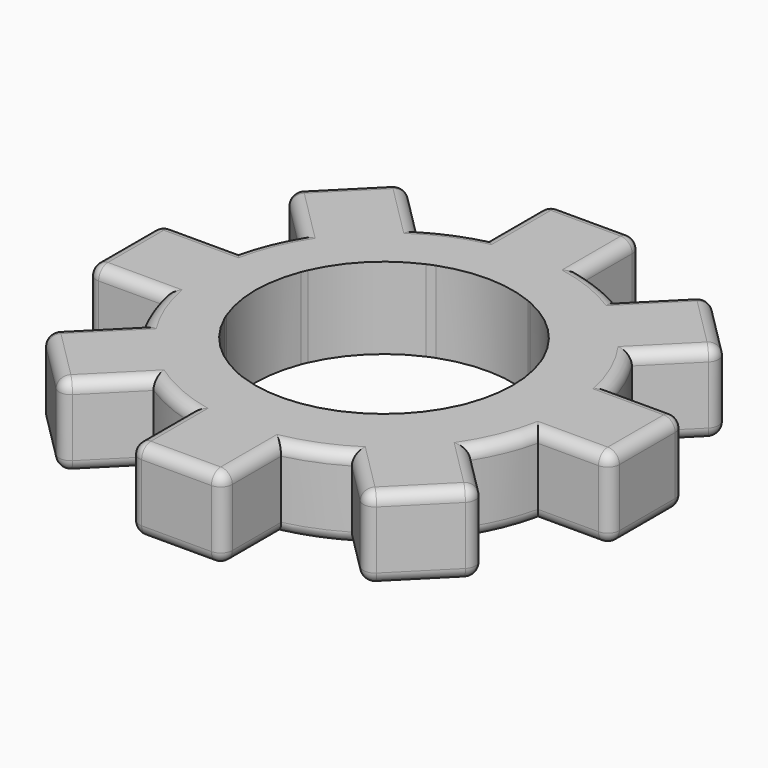
from build123d import *

# Parameters (mm, degrees)
F1_DEPTH     = 7
F2_R         = 1
F3_R         = 1
F4_T1_DEPTH  = 6
F4_T3_DEPTH  = 5
F4_T5_DEPTH  = 6
F4_T7_DEPTH  = 6
F4_T9_DEPTH  = 6
F4_T11_DEPTH = 6
F4_T13_DEPTH = 6
F4_T16_ANGLE = 90
F4_T18_ANGLE = 90
F4_T20_ANGLE = 90
F4_T22_ANGLE = 90
F4_T24_ANGLE = 90
F4_T26_ANGLE = 90
F4_T28_ANGLE = 90
F4_T30_ANGLE = 90
F4_T32_ANGLE = 90
F4_T34_ANGLE = 90
F4_T36_ANGLE = 90
F4_T38_ANGLE = 90
F4_T40_ANGLE = 90
F4_T42_ANGLE = 90
F4_T44_ANGLE = 90
F4_T46_ANGLE = 90
F4_T48_ANGLE = 90
F4_T50_ANGLE = 90
F4_T52_ANGLE = 90
F4_T54_ANGLE = 90
F4_T56_ANGLE = 90
F4_T58_ANGLE = 90
F4_T60_ANGLE = 90
F4_T62_ANGLE = 90
F4_T64_ANGLE = 90
F4_T66_ANGLE = 90
F4_T68_ANGLE = 90
F4_T70_ANGLE = 90
F4_T72_ANGLE = 90
F4_T74_ANGLE = 90
F4_T76_ANGLE = 90
F4_T78_ANGLE = 90


# Not quite as in the source:
# - a fillet or chamfer that OpenCascade refuses, or shapes differently, is made with other operations: its cross-section is extruded or revolved along the edge and cut away or added


with BuildPart() as f1:
    # F0 (on Top) → F1 (new body)
    with BuildSketch(Plane.XY):
        with BuildLine():
            Line((-18.9102605216, 13.1071560315), (-14.0960219885, 8.2929174984))
            ThreePointArc((-14.0960219885, 8.2929174984), (-11.6421815939, 11.4897849201), (-8.4893514939, 13.9999555028))
            Line((-8.4893514939, 13.9999555028), (-13.2534062721, 18.764010281))
            Line((-13.2534062721, 18.764010281), (-18.9102605216, 13.1071560315))
        make_face()
        with BuildLine():
            ThreePointArc((-8.4893514939, 13.9999555028), (-11.6421815939, 11.4897849201), (-14.0960219885, 8.2929174984))
            Line((-14.0960219885, 8.2929174984), (-10.3029473829, 4.4998428928))
            ThreePointArc((-10.3029473829, 4.4998428928), (-8.0031384218, 7.8568881812), (-4.6460931334, 10.1566971423))
            Line((-4.6460931334, 10.1566971423), (-8.4893514939, 13.9999555028))
        make_face()
        with BuildLine():
            ThreePointArc((-4, 15.9127699712), (-6.315455609, 15.1224821829), (-8.4893514939, 13.9999555028))
            Line((-8.4893514939, 13.9999555028), (-4.6460931334, 10.1566971423))
            ThreePointArc((-4.6460931334, 10.1566971423), (-4.3251030215, 10.2924612661), (-4, 10.4180581398))
            Line((-4, 10.4180581398), (-4, 15.9127699712))
        make_face()
        with BuildLine():
            ThreePointArc((4, 16.0031068635), (-0.0055323046, 16.4478649132), (-4, 15.9127699712))
            Line((-4, 15.9127699712), (-4, 10.4180581398))
            ThreePointArc((-4, 10.4180581398), (0.012449523, 11.0991456601), (4, 10.2848529747))
            Line((4, 10.2848529747), (4, 16.0031068635))
        make_face()
        with BuildLine():
            Line((-4, 22.5), (-4, 15.9127699712))
            ThreePointArc((-4, 15.9127699712), (-0.0055323046, 16.4478649132), (4, 16.0031068635))
            Line((4, 16.0031068635), (4, 22.5))
            Line((4, 22.5), (-4, 22.5))
        make_face()
        with BuildLine():
            Line((4.3022314931, 10.1566971423), (8.4085999773, 14.2630656264))
            ThreePointArc((8.4085999773, 14.2630656264), (6.2668160064, 15.2914779593), (4, 16.0031068635))
            Line((4, 16.0031068635), (4, 10.2848529747))
            ThreePointArc((4, 10.2848529747), (4.1515906147, 10.2218949458), (4.3022314931, 10.1566971423))
        make_face()
        with BuildLine():
            Line((9.9590857426, 4.4998428928), (14.1911468506, 8.7319040008))
            ThreePointArc((14.1911468506, 8.7319040008), (11.63867014, 11.8516794804), (8.4085999773, 14.2630656264))
            Line((8.4085999773, 14.2630656264), (4.3022314931, 10.1566971423))
            ThreePointArc((4.3022314931, 10.1566971423), (7.6592767815, 7.8568881812), (9.9590857426, 4.4998428928))
        make_face()
        with BuildLine():
            ThreePointArc((8.4085999773, 14.2630656264), (11.63867014, 11.8516794804), (14.1911468506, 8.7319040008))
            Line((14.1911468506, 8.7319040008), (18.5663988813, 13.1071560315))
            Line((18.5663988813, 13.1071560315), (12.9095446318, 18.764010281))
            Line((12.9095446318, 18.764010281), (8.4085999773, 14.2630656264))
        make_face()
        with BuildLine():
            Line((10.1654000803, 4), (16.2348496569, 4))
            ThreePointArc((16.2348496569, 4), (15.3980605169, 6.4458801364), (14.1911468506, 8.7319040008))
            Line((14.1911468506, 8.7319040008), (9.9590857426, 4.4998428928))
            ThreePointArc((9.9590857426, 4.4998428928), (10.0652940332, 4.2511808224), (10.1654000803, 4))
        make_face()
        with BuildLine():
            Line((10.1455068885, -4), (16.2975573812, -4))
            ThreePointArc((16.2975573812, -4), (16.6414561301, -2.0765917699), (16.7566225123, -0.126078434))
            ThreePointArc((16.7566225123, -0.126078434), (16.6256619327, 1.9533908587), (16.2348496569, 4))
            Line((16.2348496569, 4), (10.1654000803, 4))
            ThreePointArc((10.1654000803, 4), (10.7170903646, 2.0467799435), (10.9030691799, 0.0256805796))
            ThreePointArc((10.9030691799, 0.0256805796), (10.7120309499, -2.0224896254), (10.1455068885, -4))
        make_face()
        with BuildLine():
            ThreePointArc((16.7566225123, -0.126078434), (16.6414561301, -2.0765917699), (16.2975573812, -4))
            Line((16.2975573812, -4), (22.5, -4))
            Line((22.5, -4), (22.5, 4))
            Line((22.5, 4), (16.2348496569, 4))
            ThreePointArc((16.2348496569, 4), (16.6256619327, 1.9533908587), (16.7566225123, -0.126078434))
        make_face()
        with BuildLine():
            Line((9.9590857426, -4.4484817337), (14.3076564491, -8.7970524402))
            ThreePointArc((14.3076564491, -8.7970524402), (15.4916550838, -6.4769466942), (16.2975573812, -4))
            Line((16.2975573812, -4), (10.1455068885, -4))
            ThreePointArc((10.1455068885, -4), (10.0547550795, -4.2252629053), (9.9590857426, -4.4484817337))
        make_face()
        with BuildLine():
            Line((4.3022314931, -10.1053359832), (8.6006184447, -14.4037229347))
            ThreePointArc((8.6006184447, -14.4037229347), (11.7974858663, -11.9498825401), (14.3076564491, -8.7970524402))
            Line((14.3076564491, -8.7970524402), (9.9590857426, -4.4484817337))
            ThreePointArc((9.9590857426, -4.4484817337), (7.6592767815, -7.8055270221), (4.3022314931, -10.1053359832))
        make_face()
        with BuildLine():
            ThreePointArc((14.3076564491, -8.7970524402), (11.7974858663, -11.9498825401), (8.6006184447, -14.4037229347))
            Line((8.6006184447, -14.4037229347), (12.9095446318, -18.7126491219))
            Line((12.9095446318, -18.7126491219), (18.5663988813, -13.0557948724))
            Line((18.5663988813, -13.0557948724), (14.3076564491, -8.7970524402))
        make_face()
        with BuildLine():
            ThreePointArc((-4, -16.1649268392), (-0.0055323046, -16.7000217811), (4, -16.2552637315))
            Line((4, -16.2552637315), (4, -10.2334918155))
            ThreePointArc((4, -10.2334918155), (0.012449523, -11.0477845009), (-4, -10.3666969806))
            Line((-4, -10.3666969806), (-4, -16.1649268392))
        make_face()
        with BuildLine():
            Line((-4, -22.5), (4, -22.5))
            Line((4, -22.5), (4, -16.2552637315))
            ThreePointArc((4, -16.2552637315), (-0.0055323046, -16.7000217811), (-4, -16.1649268392))
            Line((-4, -16.1649268392), (-4, -22.5))
        make_face()
        with BuildLine():
            Line((4, -10.2334918155), (4, -16.2552637315))
            ThreePointArc((4, -16.2552637315), (6.369948448, -15.5025294911), (8.6006184447, -14.4037229347))
            Line((8.6006184447, -14.4037229347), (4.3022314931, -10.1053359832))
            ThreePointArc((4.3022314931, -10.1053359832), (4.1515906147, -10.1705337867), (4, -10.2334918155))
        make_face()
        with BuildLine():
            ThreePointArc((-8.6763599225, -14.1356027723), (-6.4166623661, -15.3311191003), (-4, -16.1649268392))
            Line((-4, -16.1649268392), (-4, -10.3666969806))
            ThreePointArc((-4, -10.3666969806), (-4.3251030215, -10.241100107), (-4.6460931334, -10.1053359832))
            Line((-4.6460931334, -10.1053359832), (-8.6763599225, -14.1356027723))
        make_face()
        with BuildLine():
            ThreePointArc((-14.2075215481, -8.3530558989), (-11.7961354021, -11.5831260617), (-8.6763599225, -14.1356027723))
            Line((-8.6763599225, -14.1356027723), (-4.6460931334, -10.1053359832))
            ThreePointArc((-4.6460931334, -10.1053359832), (-8.0031384218, -7.8055270221), (-10.3029473829, -4.4484817337))
            Line((-10.3029473829, -4.4484817337), (-14.2075215481, -8.3530558989))
        make_face()
        with BuildLine():
            Line((-13.2534062721, -18.7126491219), (-8.6763599225, -14.1356027723))
            ThreePointArc((-8.6763599225, -14.1356027723), (-11.7961354021, -11.5831260617), (-14.2075215481, -8.3530558989))
            Line((-14.2075215481, -8.3530558989), (-18.9102605216, -13.0557948724))
            Line((-18.9102605216, -13.0557948724), (-13.2534062721, -18.7126491219))
        make_face()
        with BuildLine():
            ThreePointArc((-15.9343123567, -4), (-15.2254289265, -6.2378204904), (-14.2075215481, -8.3530558989))
            Line((-14.2075215481, -8.3530558989), (-10.3029473829, -4.4484817337))
            ThreePointArc((-10.3029473829, -4.4484817337), (-10.3986167197, -4.2252629053), (-10.4893685287, -4))
            Line((-10.4893685287, -4), (-15.9343123567, -4))
        make_face()
        with BuildLine():
            ThreePointArc((-15.8716046323, 4), (-16.3928683144, 0.0038401412), (-15.9343123567, -4))
            Line((-15.9343123567, -4), (-10.4893685287, -4))
            ThreePointArc((-10.4893685287, -4), (-11.2468965796, -0.0018589727), (-10.5092617205, 4))
            Line((-10.5092617205, 4), (-15.8716046323, 4))
        make_face()
        with BuildLine():
            Line((-22.5, -4), (-15.9343123567, -4))
            ThreePointArc((-15.9343123567, -4), (-16.3928683144, 0.0038401412), (-15.8716046323, 4))
            Line((-15.8716046323, 4), (-22.5, 4))
            Line((-22.5, 4), (-22.5, -4))
        make_face()
        with BuildLine():
            ThreePointArc((-14.0960219885, 8.2929174984), (-15.1349609466, 6.2089745371), (-15.8716046323, 4))
            Line((-15.8716046323, 4), (-10.5092617205, 4))
            ThreePointArc((-10.5092617205, 4), (-10.4091556734, 4.2511808224), (-10.3029473829, 4.4998428928))
            Line((-10.3029473829, 4.4998428928), (-14.0960219885, 8.2929174984))
        make_face()
    extrude(amount=F1_DEPTH)

    # F2
    f2_edges = [f1.edges().sort_by_distance(p)[0] for p in [
        (-10.871379, 16.381983, 7),
        (-6.315456, 15.122482, 7),
        (-4, 19.206385, 7),
        (4, 19.251553, 7),
        (6.266816, 15.291478, 7),
        (10.659072, 16.513538, 7),
        (16.378773, 10.91953, 7),
        (19.367425, 4, 7),
        (19.398779, -4, 7),
        (15.398061, 6.44588, 7),
        (15.491655, -6.476947, 7),
        (16.437028, -10.926424, 7),
        (10.755082, -16.558186, 7),
        (6.369948, -15.502529, 7),
        (4, -19.377632, 7),
        (-4, -19.332463, 7),
        (-6.416662, -15.331119, 7),
        (-10.964883, -16.424126, 7),
        (-16.558891, -10.704425, 7),
        (-15.225429, -6.23782, 7),
        (-19.217156, -4, 7),
        (-19.185802, 4, 7),
        (-15.134961, 6.208975, 7),
        (-16.503141, 10.700037, 7),
    ]]
    fillet(f2_edges, radius=F2_R)

    # F3
    f3_edges = [f1.edges().sort_by_distance(p)[0] for p in [
        (16.437028, -10.926424, 0),
        (10.755082, -16.558186, 0),
        (15.491655, -6.476947, 0),
        (6.369948, -15.502529, 0),
        (4, -19.377632, 0),
        (-4, -19.332463, 0),
        (-6.416662, -15.331119, 0),
        (-10.964883, -16.424126, 0),
        (-16.558891, -10.704425, 0),
        (-15.225429, -6.23782, 0),
        (-19.217156, -4, 0),
        (-19.185802, 4, 0),
        (-15.134961, 6.208975, 0),
        (-16.503141, 10.700037, 0),
        (-10.871379, 16.381983, 0),
        (-6.315456, 15.122482, 0),
        (-4, 19.206385, 0),
        (4, 19.251553, 0),
        (6.266816, 15.291478, 0),
        (10.659072, 16.513538, 0),
        (16.378773, 10.91953, 0),
        (15.398061, 6.44588, 0),
        (19.367425, 4, 0),
        (19.398779, -4, 0),
    ]]
    fillet(f3_edges, radius=F3_R)

    # F4: fillet of radius 1 on 64 edges, made by hand

    # F4_s2 → F4_t1 (cut)
    with BuildSketch(Plane(origin=(-2.1944454638, -2.1944454638, 0), x_dir=(0, 0, 1), z_dir=(0.7071067812, 0.7071067812, 0))):
        with BuildLine():
            ThreePointArc((7, 21.3602676392), (6.7071067812, 22.0673744204), (6, 22.3602676392))
            Line((6, 22.3602676392), (7, 22.3602676392))
            Line((7, 22.3602676392), (7, 21.3602676392))
        make_face()
        with BuildLine():
            ThreePointArc((0, 21.3602676392), (0.2928932188, 22.0673744204), (1, 22.3602676392))
            Line((1, 22.3602676392), (0, 22.3602676392))
            Line((0, 22.3602676392), (0, 21.3602676392))
        make_face()
    extrude(amount=F4_T1_DEPTH, mode=Mode.SUBTRACT)

    # F4_s4 → F4_t3 (cut)
    with BuildSketch(Plane.XY.offset(1)):
        with BuildLine():
            ThreePointArc((13.616651413, -18.0055423407), (12.9095446318, -18.2984355595), (12.2024378507, -18.0055423407))
            Line((12.2024378507, -18.0055423407), (12.9095446318, -18.7126491219))
            Line((12.9095446318, -18.7126491219), (13.616651413, -18.0055423407))
        make_face()
        with BuildLine():
            ThreePointArc((17.8592921001, -13.7629016536), (18.152185319, -13.0557948724), (17.8592921001, -12.3486880912))
            Line((17.8592921001, -12.3486880912), (18.5663988813, -13.0557948724))
            Line((18.5663988813, -13.0557948724), (17.8592921001, -13.7629016536))
        make_face()
        with BuildLine():
            ThreePointArc((-3, -22.5), (-3.7071067812, -22.2071067812), (-4, -21.5))
            Line((-4, -21.5), (-4, -22.5))
            Line((-4, -22.5), (-3, -22.5))
        make_face()
        with BuildLine():
            ThreePointArc((3, -22.5), (3.7071067812, -22.2071067812), (4, -21.5))
            Line((4, -21.5), (4, -22.5))
            Line((4, -22.5), (3, -22.5))
        make_face()
        with BuildLine():
            ThreePointArc((-13.9605130533, -18.0055423407), (-13.2534062721, -18.2984355595), (-12.5462994909, -18.0055423407))
            Line((-12.5462994909, -18.0055423407), (-13.2534062721, -18.7126491219))
            Line((-13.2534062721, -18.7126491219), (-13.9605130533, -18.0055423407))
        make_face()
        with BuildLine():
            ThreePointArc((-18.2031537404, -13.7629016536), (-18.4960469592, -13.0557948724), (-18.2031537404, -12.3486880912))
            Line((-18.2031537404, -12.3486880912), (-18.9102605216, -13.0557948724))
            Line((-18.9102605216, -13.0557948724), (-18.2031537404, -13.7629016536))
        make_face()
        with BuildLine():
            ThreePointArc((-22.5, 3), (-22.2071067812, 3.7071067812), (-21.5, 4))
            Line((-21.5, 4), (-22.5, 4))
            Line((-22.5, 4), (-22.5, 3))
        make_face()
        with BuildLine():
            ThreePointArc((-22.5, -3), (-22.2071067812, -3.7071067812), (-21.5, -4))
            Line((-21.5, -4), (-22.5, -4))
            Line((-22.5, -4), (-22.5, -3))
        make_face()
        with BuildLine():
            ThreePointArc((-18.2031537404, 13.8142628127), (-18.4960469592, 13.1071560315), (-18.2031537404, 12.4000492503))
            Line((-18.2031537404, 12.4000492503), (-18.9102605216, 13.1071560315))
            Line((-18.9102605216, 13.1071560315), (-18.2031537404, 13.8142628127))
        make_face()
        with BuildLine():
            ThreePointArc((-13.9605130532, 18.0569034998), (-13.2534062721, 18.3497967186), (-12.5462994909, 18.0569034998))
            Line((-12.5462994909, 18.0569034998), (-13.2534062721, 18.764010281))
            Line((-13.2534062721, 18.764010281), (-13.9605130532, 18.0569034998))
        make_face()
        with BuildLine():
            ThreePointArc((3, 22.5), (3.7071067812, 22.2071067812), (4, 21.5))
            Line((4, 21.5), (4, 22.5))
            Line((4, 22.5), (3, 22.5))
        make_face()
        with BuildLine():
            ThreePointArc((-3, 22.5), (-3.7071067812, 22.2071067812), (-4, 21.5))
            Line((-4, 21.5), (-4, 22.5))
            Line((-4, 22.5), (-3, 22.5))
        make_face()
        with BuildLine():
            ThreePointArc((17.8592921001, 13.8142628127), (18.152185319, 13.1071560315), (17.8592921001, 12.4000492503))
            Line((17.8592921001, 12.4000492503), (18.5663988813, 13.1071560315))
            Line((18.5663988813, 13.1071560315), (17.8592921001, 13.8142628127))
        make_face()
        with BuildLine():
            ThreePointArc((13.616651413, 18.0569034998), (12.9095446318, 18.3497967186), (12.2024378507, 18.0569034998))
            Line((12.2024378507, 18.0569034998), (12.9095446318, 18.764010281))
            Line((12.9095446318, 18.764010281), (13.616651413, 18.0569034998))
        make_face()
        with BuildLine():
            ThreePointArc((22.5, 3), (22.2071067812, 3.7071067812), (21.5, 4))
            Line((21.5, 4), (22.5, 4))
            Line((22.5, 4), (22.5, 3))
        make_face()
        with BuildLine():
            ThreePointArc((22.5, -3), (22.2071067812, -3.7071067812), (21.5, -4))
            Line((21.5, -4), (22.5, -4))
            Line((22.5, -4), (22.5, -3))
        make_face()
    extrude(amount=F4_T3_DEPTH, mode=Mode.SUBTRACT)

    # F4_s6 → F4_t5 (cut)
    with BuildSketch(Plane.YZ.offset(-3)):
        with BuildLine():
            ThreePointArc((-21.5, 7), (-22.2071067812, 6.7071067812), (-22.5, 6))
            Line((-22.5, 6), (-22.5, 7))
            Line((-22.5, 7), (-21.5, 7))
        make_face()
        with BuildLine():
            ThreePointArc((-21.5, 0), (-22.2071067812, 0.2928932188), (-22.5, 1))
            Line((-22.5, 1), (-22.5, 0))
            Line((-22.5, 0), (-21.5, 0))
        make_face()
        with BuildLine():
            ThreePointArc((21.5, 7), (22.2071067812, 6.7071067812), (22.5, 6))
            Line((22.5, 6), (22.5, 7))
            Line((22.5, 7), (21.5, 7))
        make_face()
        with BuildLine():
            ThreePointArc((21.5, 0), (22.2071067812, 0.2928932188), (22.5, 1))
            Line((22.5, 1), (22.5, 0))
            Line((22.5, 0), (21.5, 0))
        make_face()
    extrude(amount=F4_T5_DEPTH, mode=Mode.SUBTRACT)

    # F4_s8 → F4_t7 (cut)
    with BuildSketch(Plane(origin=(-2.2201260434, 2.2201260434, 0), x_dir=(0, 0, 1), z_dir=(0.7071067812, -0.7071067812, 0))):
        with BuildLine():
            ThreePointArc((7, 21.6034145368), (6.7071067812, 22.310521318), (6, 22.6034145368))
            Line((6, 22.6034145368), (7, 22.6034145368))
            Line((7, 22.6034145368), (7, 21.6034145368))
        make_face()
        with BuildLine():
            ThreePointArc((0, 21.6034145368), (0.2928932188, 22.310521318), (1, 22.6034145368))
            Line((1, 22.6034145368), (0, 22.6034145368))
            Line((0, 22.6034145368), (0, 21.6034145368))
        make_face()
    extrude(amount=F4_T7_DEPTH, mode=Mode.SUBTRACT)

    # F4_s10 → F4_t9 (cut)
    with BuildSketch(Plane.XZ.offset(-3)):
        with BuildLine():
            ThreePointArc((-21.5, 7), (-22.2071067812, 6.7071067812), (-22.5, 6))
            Line((-22.5, 6), (-22.5, 7))
            Line((-22.5, 7), (-21.5, 7))
        make_face()
        with BuildLine():
            ThreePointArc((-21.5, 0), (-22.2071067812, 0.2928932188), (-22.5, 1))
            Line((-22.5, 1), (-22.5, 0))
            Line((-22.5, 0), (-21.5, 0))
        make_face()
        with BuildLine():
            ThreePointArc((21.5, 0), (22.2071067812, 0.2928932188), (22.5, 1))
            Line((22.5, 1), (22.5, 0))
            Line((22.5, 0), (21.5, 0))
        make_face()
        with BuildLine():
            ThreePointArc((21.5, 7), (22.2071067812, 6.7071067812), (22.5, 6))
            Line((22.5, 6), (22.5, 7))
            Line((22.5, 7), (21.5, 7))
        make_face()
    extrude(amount=F4_T9_DEPTH, mode=Mode.SUBTRACT)

    # F4_s12 → F4_t11 (cut)
    with BuildSketch(Plane(origin=(2.0481952233, 2.0481952233, 0), x_dir=(0, 0, 1), z_dir=(-0.7071067812, -0.7071067812, 0))):
        with BuildLine():
            ThreePointArc((6, 22.6397323608), (6.7071067812, 22.3468391419), (7, 21.6397323608))
            Line((7, 21.6397323608), (7, 22.6397323608))
            Line((7, 22.6397323608), (6, 22.6397323608))
        make_face()
        with BuildLine():
            ThreePointArc((1, 22.6397323608), (0.2928932188, 22.3468391419), (0, 21.6397323608))
            Line((0, 21.6397323608), (0, 22.6397323608))
            Line((0, 22.6397323608), (1, 22.6397323608))
        make_face()
    extrude(amount=F4_T11_DEPTH, mode=Mode.SUBTRACT)

    # F4_s14 → F4_t13 (cut)
    with BuildSketch(Plane(origin=(2.0225146437, -2.0225146437, 0), x_dir=(0, 0, 1), z_dir=(-0.7071067812, 0.7071067812, 0))):
        with BuildLine():
            ThreePointArc((0, 21.3965854632), (0.2928932188, 22.1036922443), (1, 22.3965854632))
            Line((1, 22.3965854632), (0, 22.3965854632))
            Line((0, 22.3965854632), (0, 21.3965854632))
        make_face()
        with BuildLine():
            ThreePointArc((7, 21.3965854632), (6.7071067812, 22.1036922443), (6, 22.3965854632))
            Line((6, 22.3965854632), (7, 22.3965854632))
            Line((7, 22.3965854632), (7, 21.3965854632))
        make_face()
    extrude(amount=F4_T13_DEPTH, mode=Mode.SUBTRACT)

    # F4_s15 → F4_t16 (revolve, cut)
    with BuildSketch(Plane.XY.offset(1)):
        with BuildLine():
            ThreePointArc((-13.9605130532, 18.0569034998), (-13.2534062721, 18.3497967186), (-12.5462994909, 18.0569034998))
            Line((-12.5462994909, 18.0569034998), (-13.2534062721, 18.764010281))
            Line((-13.2534062721, 18.764010281), (-13.9605130532, 18.0569034998))
        make_face()
    revolve(axis=Axis((-13.9605130533, 18.0569034998, 1), (-0.7071067812, 0.7071067812, 0)), revolution_arc=F4_T16_ANGLE, mode=Mode.SUBTRACT)

    # F4_s17 → F4_t18 (revolve, cut)
    with BuildSketch(Plane.XY.offset(6)):
        with BuildLine():
            ThreePointArc((-13.9605130532, 18.0569034998), (-13.2534062721, 18.3497967186), (-12.5462994909, 18.0569034998))
            Line((-12.5462994909, 18.0569034998), (-13.2534062721, 18.764010281))
            Line((-13.2534062721, 18.764010281), (-13.9605130532, 18.0569034998))
        make_face()
    revolve(axis=Axis((-13.9605130533, 18.0569034998, 6), (0.7071067812, -0.7071067812, 0)), revolution_arc=F4_T18_ANGLE, mode=Mode.SUBTRACT)

    # F4_s19 → F4_t20 (revolve, cut)
    with BuildSketch(Plane(origin=(-2.1944454638, -2.1944454638, 0), x_dir=(0, 0, 1), z_dir=(0.7071067812, 0.7071067812, 0))):
        with BuildLine():
            ThreePointArc((1, -22.6397323608), (0.2928932188, -22.3468391419), (0, -21.6397323608))
            Line((0, -21.6397323608), (0, -22.6397323608))
            Line((0, -22.6397323608), (1, -22.6397323608))
        make_face()
    revolve(axis=Axis((-18.2031537404, 13.8142628127, 1), (-0.7071067812, 0.7071067812, 0)), revolution_arc=F4_T20_ANGLE, mode=Mode.SUBTRACT)

    # F4_s21 → F4_t22 (revolve, cut)
    with BuildSketch(Plane.XY.offset(6)):
        with BuildLine():
            ThreePointArc((-18.2031537404, 13.8142628127), (-18.4960469592, 13.1071560315), (-18.2031537404, 12.4000492503))
            Line((-18.2031537404, 12.4000492503), (-18.9102605216, 13.1071560315))
            Line((-18.9102605216, 13.1071560315), (-18.2031537404, 13.8142628127))
        make_face()
    revolve(axis=Axis((-18.2031537404, 13.8142628127, 6), (-0.7071067812, 0.7071067812, 0)), revolution_arc=F4_T22_ANGLE, mode=Mode.SUBTRACT)

    # F4_s23 → F4_t24 (revolve, cut)
    with BuildSketch(Plane.YZ.offset(-3)):
        with BuildLine():
            ThreePointArc((21.5, 0), (22.2071067812, 0.2928932188), (22.5, 1))
            Line((22.5, 1), (22.5, 0))
            Line((22.5, 0), (21.5, 0))
        make_face()
    revolve(axis=Axis((-3, 22.5, 1), (0, 1, 0)), revolution_arc=F4_T24_ANGLE, mode=Mode.SUBTRACT)

    # F4_s25 → F4_t26 (revolve, cut)
    with BuildSketch(Plane.XZ.offset(-3)):
        with BuildLine():
            ThreePointArc((-21.5, 0), (-22.2071067812, 0.2928932188), (-22.5, 1))
            Line((-22.5, 1), (-22.5, 0))
            Line((-22.5, 0), (-21.5, 0))
        make_face()
    revolve(axis=Axis((-22.5, 3, 1), (1, 0, 0)), revolution_arc=F4_T26_ANGLE, mode=Mode.SUBTRACT)

    # F4_s27 → F4_t28 (revolve, cut)
    with BuildSketch(Plane.YZ.offset(3)):
        with BuildLine():
            ThreePointArc((22.5, 1), (22.2071067812, 0.2928932188), (21.5, 0))
            Line((21.5, 0), (22.5, 0))
            Line((22.5, 0), (22.5, 1))
        make_face()
    revolve(axis=Axis((3, 22.5, 1), (0, -1, 0)), revolution_arc=F4_T28_ANGLE, mode=Mode.SUBTRACT)

    # F4_s29 → F4_t30 (revolve, cut)
    with BuildSketch(Plane.XY.offset(6)):
        with BuildLine():
            ThreePointArc((3, 22.5), (3.7071067812, 22.2071067812), (4, 21.5))
            Line((4, 21.5), (4, 22.5))
            Line((4, 22.5), (3, 22.5))
        make_face()
    revolve(axis=Axis((3, 22.5, 6), (0, -1, 0)), revolution_arc=F4_T30_ANGLE, mode=Mode.SUBTRACT)

    # F4_s31 → F4_t32 (revolve, cut)
    with BuildSketch(Plane.XY.offset(6)):
        with BuildLine():
            ThreePointArc((-3, 22.5), (-3.7071067812, 22.2071067812), (-4, 21.5))
            Line((-4, 21.5), (-4, 22.5))
            Line((-4, 22.5), (-3, 22.5))
        make_face()
    revolve(axis=Axis((-3, 22.5, 6), (0, 1, 0)), revolution_arc=F4_T32_ANGLE, mode=Mode.SUBTRACT)

    # F4_s33 → F4_t34 (revolve, cut)
    with BuildSketch(Plane.XY.offset(6)):
        with BuildLine():
            ThreePointArc((-22.5, 3), (-22.2071067812, 3.7071067812), (-21.5, 4))
            Line((-21.5, 4), (-22.5, 4))
            Line((-22.5, 4), (-22.5, 3))
        make_face()
    revolve(axis=Axis((-22.5, 3, 6), (1, 0, 0)), revolution_arc=F4_T34_ANGLE, mode=Mode.SUBTRACT)

    # F4_s35 → F4_t36 (revolve, cut)
    with BuildSketch(Plane.XZ.offset(3)):
        with BuildLine():
            ThreePointArc((-22.5, 1), (-22.2071067812, 0.2928932188), (-21.5, 0))
            Line((-21.5, 0), (-22.5, 0))
            Line((-22.5, 0), (-22.5, 1))
        make_face()
    revolve(axis=Axis((-22.5, -3, 1), (-1, 0, 0)), revolution_arc=F4_T36_ANGLE, mode=Mode.SUBTRACT)

    # F4_s37 → F4_t38 (revolve, cut)
    with BuildSketch(Plane.XY.offset(6)):
        with BuildLine():
            ThreePointArc((-22.5, -3), (-22.2071067812, -3.7071067812), (-21.5, -4))
            Line((-21.5, -4), (-22.5, -4))
            Line((-22.5, -4), (-22.5, -3))
        make_face()
    revolve(axis=Axis((-22.5, -3, 6), (-1, 0, 0)), revolution_arc=F4_T38_ANGLE, mode=Mode.SUBTRACT)

    # F4_s39 → F4_t40 (revolve, cut)
    with BuildSketch(Plane(origin=(-2.2201260434, 2.2201260434, 0), x_dir=(0, 0, 1), z_dir=(0.7071067812, -0.7071067812, 0))):
        with BuildLine():
            ThreePointArc((0, -21.3965854632), (0.2928932188, -22.1036922443), (1, -22.3965854632))
            Line((1, -22.3965854632), (0, -22.3965854632))
            Line((0, -22.3965854632), (0, -21.3965854632))
        make_face()
    revolve(axis=Axis((13.616651413, 18.0569034998, 1), (0.7071067812, 0.7071067812, 0)), revolution_arc=F4_T40_ANGLE, mode=Mode.SUBTRACT)

    # F4_s41 → F4_t42 (revolve, cut)
    with BuildSketch(Plane(origin=(-2.2201260434, 2.2201260434, 0), x_dir=(0, 0, 1), z_dir=(0.7071067812, -0.7071067812, 0))):
        with BuildLine():
            ThreePointArc((0, 21.6034145368), (0.2928932188, 22.310521318), (1, 22.6034145368))
            Line((1, 22.6034145368), (0, 22.6034145368))
            Line((0, 22.6034145368), (0, 21.6034145368))
        make_face()
    revolve(axis=Axis((-18.2031537404, -13.7629016536, 1), (0.7071067812, 0.7071067812, 0)), revolution_arc=F4_T42_ANGLE, mode=Mode.SUBTRACT)

    # F4_s43 → F4_t44 (revolve, cut)
    with BuildSketch(Plane(origin=(2.0225146437, -2.0225146437, 0), x_dir=(0, 0, 1), z_dir=(-0.7071067812, 0.7071067812, 0))):
        with BuildLine():
            ThreePointArc((1, 22.3965854632), (0.2928932188, 22.1036922443), (0, 21.3965854632))
            Line((0, 21.3965854632), (0, 22.3965854632))
            Line((0, 22.3965854632), (1, 22.3965854632))
        make_face()
    revolve(axis=Axis((17.8592921001, 13.8142628127, 1), (-0.7071067812, -0.7071067812, 0)), revolution_arc=F4_T44_ANGLE, mode=Mode.SUBTRACT)

    # F4_s45 → F4_t46 (revolve, cut)
    with BuildSketch(Plane.XY.offset(6)):
        with BuildLine():
            ThreePointArc((17.8592921001, 13.8142628127), (18.152185319, 13.1071560315), (17.8592921001, 12.4000492503))
            Line((17.8592921001, 12.4000492503), (18.5663988813, 13.1071560315))
            Line((18.5663988813, 13.1071560315), (17.8592921001, 13.8142628127))
        make_face()
    revolve(axis=Axis((17.8592921001, 13.8142628127, 6), (-0.7071067812, -0.7071067812, 0)), revolution_arc=F4_T46_ANGLE, mode=Mode.SUBTRACT)

    # F4_s47 → F4_t48 (revolve, cut)
    with BuildSketch(Plane.XY.offset(6)):
        with BuildLine():
            ThreePointArc((13.616651413, 18.0569034998), (12.9095446318, 18.3497967186), (12.2024378507, 18.0569034998))
            Line((12.2024378507, 18.0569034998), (12.9095446318, 18.764010281))
            Line((12.9095446318, 18.764010281), (13.616651413, 18.0569034998))
        make_face()
    revolve(axis=Axis((13.616651413, 18.0569034998, 6), (0.7071067812, 0.7071067812, 0)), revolution_arc=F4_T48_ANGLE, mode=Mode.SUBTRACT)

    # F4_s49 → F4_t50 (revolve, cut)
    with BuildSketch(Plane.XY.offset(6)):
        with BuildLine():
            ThreePointArc((-18.2031537404, -13.7629016536), (-18.4960469592, -13.0557948724), (-18.2031537404, -12.3486880912))
            Line((-18.2031537404, -12.3486880912), (-18.9102605216, -13.0557948724))
            Line((-18.9102605216, -13.0557948724), (-18.2031537404, -13.7629016536))
        make_face()
    revolve(axis=Axis((-18.2031537404, -13.7629016536, 6), (0.7071067812, 0.7071067812, 0)), revolution_arc=F4_T50_ANGLE, mode=Mode.SUBTRACT)

    # F4_s51 → F4_t52 (revolve, cut)
    with BuildSketch(Plane(origin=(2.0225146437, -2.0225146437, 0), x_dir=(0, 0, 1), z_dir=(-0.7071067812, 0.7071067812, 0))):
        with BuildLine():
            ThreePointArc((1, -22.6034145368), (0.2928932188, -22.310521318), (0, -21.6034145368))
            Line((0, -21.6034145368), (0, -22.6034145368))
            Line((0, -22.6034145368), (1, -22.6034145368))
        make_face()
    revolve(axis=Axis((-13.9605130532, -18.0055423407, 1), (-0.7071067812, -0.7071067812, 0)), revolution_arc=F4_T52_ANGLE, mode=Mode.SUBTRACT)

    # F4_s53 → F4_t54 (revolve, cut)
    with BuildSketch(Plane.XY.offset(6)):
        with BuildLine():
            ThreePointArc((-13.9605130532, -18.0055423407), (-13.2534062721, -18.2984355595), (-12.5462994909, -18.0055423407))
            Line((-12.5462994909, -18.0055423407), (-13.2534062721, -18.7126491219))
            Line((-13.2534062721, -18.7126491219), (-13.9605130532, -18.0055423407))
        make_face()
    revolve(axis=Axis((-13.9605130532, -18.0055423407, 6), (-0.7071067812, -0.7071067812, 0)), revolution_arc=F4_T54_ANGLE, mode=Mode.SUBTRACT)

    # F4_s55 → F4_t56 (revolve, cut)
    with BuildSketch(Plane.XZ.offset(-3)):
        with BuildLine():
            ThreePointArc((21.5, 0), (22.2071067812, 0.2928932188), (22.5, 1))
            Line((22.5, 1), (22.5, 0))
            Line((22.5, 0), (21.5, 0))
        make_face()
    revolve(axis=Axis((22.5, 3, 1), (1, 0, 0)), revolution_arc=F4_T56_ANGLE, mode=Mode.SUBTRACT)

    # F4_s57 → F4_t58 (revolve, cut)
    with BuildSketch(Plane.YZ.offset(-3)):
        with BuildLine():
            ThreePointArc((-21.5, 0), (-22.2071067812, 0.2928932188), (-22.5, 1))
            Line((-22.5, 1), (-22.5, 0))
            Line((-22.5, 0), (-21.5, 0))
        make_face()
    revolve(axis=Axis((-3, -22.5, 1), (0, 1, 0)), revolution_arc=F4_T58_ANGLE, mode=Mode.SUBTRACT)

    # F4_s59 → F4_t60 (revolve, cut)
    with BuildSketch(Plane.XZ.offset(3)):
        with BuildLine():
            ThreePointArc((22.5, 1), (22.2071067812, 0.2928932188), (21.5, 0))
            Line((21.5, 0), (22.5, 0))
            Line((22.5, 0), (22.5, 1))
        make_face()
    revolve(axis=Axis((22.5, -3, 1), (-1, 0, 0)), revolution_arc=F4_T60_ANGLE, mode=Mode.SUBTRACT)

    # F4_s61 → F4_t62 (revolve, cut)
    with BuildSketch(Plane.XY.offset(6)):
        with BuildLine():
            ThreePointArc((22.5, -3), (22.2071067812, -3.7071067812), (21.5, -4))
            Line((21.5, -4), (22.5, -4))
            Line((22.5, -4), (22.5, -3))
        make_face()
    revolve(axis=Axis((22.5, -3, 6), (-1, 0, 0)), revolution_arc=F4_T62_ANGLE, mode=Mode.SUBTRACT)

    # F4_s63 → F4_t64 (revolve, cut)
    with BuildSketch(Plane.XY.offset(6)):
        with BuildLine():
            ThreePointArc((22.5, 3), (22.2071067812, 3.7071067812), (21.5, 4))
            Line((21.5, 4), (22.5, 4))
            Line((22.5, 4), (22.5, 3))
        make_face()
    revolve(axis=Axis((22.5, 3, 6), (1, 0, 0)), revolution_arc=F4_T64_ANGLE, mode=Mode.SUBTRACT)

    # F4_s65 → F4_t66 (revolve, cut)
    with BuildSketch(Plane.XY.offset(6)):
        with BuildLine():
            ThreePointArc((-3, -22.5), (-3.7071067812, -22.2071067812), (-4, -21.5))
            Line((-4, -21.5), (-4, -22.5))
            Line((-4, -22.5), (-3, -22.5))
        make_face()
    revolve(axis=Axis((-3, -22.5, 6), (0, 1, 0)), revolution_arc=F4_T66_ANGLE, mode=Mode.SUBTRACT)

    # F4_s67 → F4_t68 (revolve, cut)
    with BuildSketch(Plane.YZ.offset(3)):
        with BuildLine():
            ThreePointArc((-22.5, 1), (-22.2071067812, 0.2928932188), (-21.5, 0))
            Line((-21.5, 0), (-22.5, 0))
            Line((-22.5, 0), (-22.5, 1))
        make_face()
    revolve(axis=Axis((3, -22.5, 1), (0, -1, 0)), revolution_arc=F4_T68_ANGLE, mode=Mode.SUBTRACT)

    # F4_s69 → F4_t70 (revolve, cut)
    with BuildSketch(Plane.XY.offset(6)):
        with BuildLine():
            ThreePointArc((3, -22.5), (3.7071067812, -22.2071067812), (4, -21.5))
            Line((4, -21.5), (4, -22.5))
            Line((4, -22.5), (3, -22.5))
        make_face()
    revolve(axis=Axis((3, -22.5, 6), (0, -1, 0)), revolution_arc=F4_T70_ANGLE, mode=Mode.SUBTRACT)

    # F4_s71 → F4_t72 (revolve, cut)
    with BuildSketch(Plane(origin=(2.0481952233, 2.0481952233, 0), x_dir=(0, 0, 1), z_dir=(-0.7071067812, -0.7071067812, 0))):
        with BuildLine():
            ThreePointArc((0, -21.3602676392), (0.2928932188, -22.0673744204), (1, -22.3602676392))
            Line((1, -22.3602676392), (0, -22.3602676392))
            Line((0, -22.3602676392), (0, -21.3602676392))
        make_face()
    revolve(axis=Axis((17.8592921001, -13.7629016536, 1), (0.7071067812, -0.7071067812, 0)), revolution_arc=F4_T72_ANGLE, mode=Mode.SUBTRACT)

    # F4_s73 → F4_t74 (revolve, cut)
    with BuildSketch(Plane(origin=(-2.1944454638, -2.1944454638, 0), x_dir=(0, 0, 1), z_dir=(0.7071067812, 0.7071067812, 0))):
        with BuildLine():
            ThreePointArc((0, 21.3602676392), (0.2928932188, 22.0673744204), (1, 22.3602676392))
            Line((1, 22.3602676392), (0, 22.3602676392))
            Line((0, 22.3602676392), (0, 21.3602676392))
        make_face()
    revolve(axis=Axis((13.616651413, -18.0055423407, 1), (-0.7071067812, 0.7071067812, 0)), revolution_arc=F4_T74_ANGLE, mode=Mode.SUBTRACT)

    # F4_s75 → F4_t76 (revolve, cut)
    with BuildSketch(Plane.XY.offset(6)):
        with BuildLine():
            ThreePointArc((13.616651413, -18.0055423407), (12.9095446318, -18.2984355595), (12.2024378507, -18.0055423407))
            Line((12.2024378507, -18.0055423407), (12.9095446318, -18.7126491219))
            Line((12.9095446318, -18.7126491219), (13.616651413, -18.0055423407))
        make_face()
    revolve(axis=Axis((13.616651413, -18.0055423407, 6), (-0.7071067812, 0.7071067812, 0)), revolution_arc=F4_T76_ANGLE, mode=Mode.SUBTRACT)

    # F4_s77 → F4_t78 (revolve, cut)
    with BuildSketch(Plane.XY.offset(6)):
        with BuildLine():
            ThreePointArc((17.8592921001, -13.7629016536), (18.152185319, -13.0557948724), (17.8592921001, -12.3486880912))
            Line((17.8592921001, -12.3486880912), (18.5663988813, -13.0557948724))
            Line((18.5663988813, -13.0557948724), (17.8592921001, -13.7629016536))
        make_face()
    revolve(axis=Axis((17.8592921001, -13.7629016536, 6), (0.7071067812, -0.7071067812, 0)), revolution_arc=F4_T78_ANGLE, mode=Mode.SUBTRACT)


solid = f1.part
